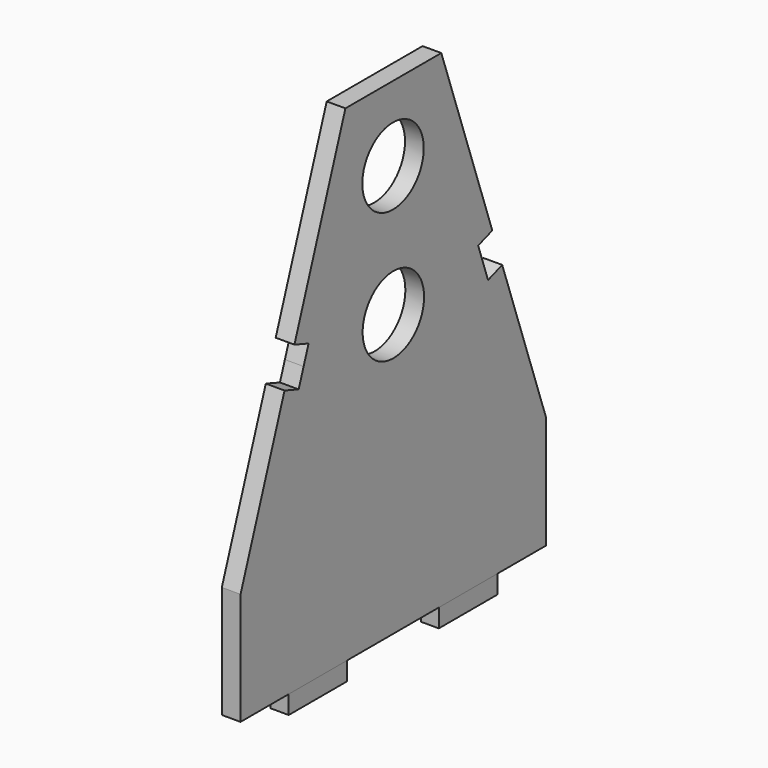
from build123d import *

# Parameters (mm, degrees)
F0_W     = 5
F0_H     = 102
F1_DEPTH = 130
F2_SIZE2 = 100
F2_SIZE  = 35
F4_W     = 4.8
F4_H     = 19.5
F5_DEPTH = 5
F6_D     = 20.5
F7_D     = 20.5
F8_DEPTH = 25


# Not quite as in the source:
# - a feature names something its author has since deleted; it is built from what else it names


with BuildPart() as f1:
    # F0 (on Top) → F1 (new body)
    with BuildSketch(Plane.XY):
        with Locations((2.5, 0.1111116846)):
            Rectangle(F0_W, F0_H)
    extrude(amount=F1_DEPTH)

    # F2
    f2_edges = [f1.edges().sort_by_distance(p)[0] for p in [
        (2.5, -50.888888, 130),
        (2.5, 51.111112, 130),
    ]]
    f2_side = f1.faces().sort_by_distance((2.5, 0.111112, 130))[0]
    chamfer(f2_edges, length=F2_SIZE, length2=F2_SIZE2, reference=f2_side)

    # F4 (on face) → F5 (join)
    with BuildSketch(Plane(origin=(0, 0, 0), x_dir=(1, 0, 0), z_dir=(0, 0, -1))):
        with Locations((2.5, -25.1611116846)):
            Rectangle(F4_W, F4_H)
        with Locations((2.5, 24.9388883154)):
            Rectangle(F4_W, F4_H)
    extrude(amount=F5_DEPTH)

    # F6 (through all)
    with Locations(Plane(origin=(0, 0, 0), x_dir=(0, -1, 0), z_dir=(-1, 0, 0))):
        with Locations((-0.1111116846, 75)):
            Hole(F6_D / 2)

    # F7 (through all)
    with Locations(Plane(origin=(0, 0, 0), x_dir=(0, -1, 0), z_dir=(-1, 0, 0))):
        with Locations((0, 110)):
            Hole(F7_D / 2)

    # F3 (on face) → F8 (cut)
    with BuildSketch(Plane(origin=(0, 0, 0), x_dir=(0, -1, 0), z_dir=(-1, 0, 0))):
        Polygon((-28.4119545359, 79.7192917818), (-33.1312463177, 81.3710439055), (-36.434750565, 71.9324603418), (-31.7154587832, 70.2807082182), (-30.0637066595, 75), align=None)
        Polygon((28.1897311666, 79.7192917818), (29.8414832903, 75), (34.5607750721, 76.6517521236), (32.9090229484, 81.3710439055), align=None)
        Polygon((34.5607750721, 76.6517521236), (29.8414832903, 75), (31.4932354139, 70.2807082182), (36.2125271957, 71.9324603418), align=None)
    extrude(amount=-F8_DEPTH, mode=Mode.SUBTRACT)


solid = f1.part
